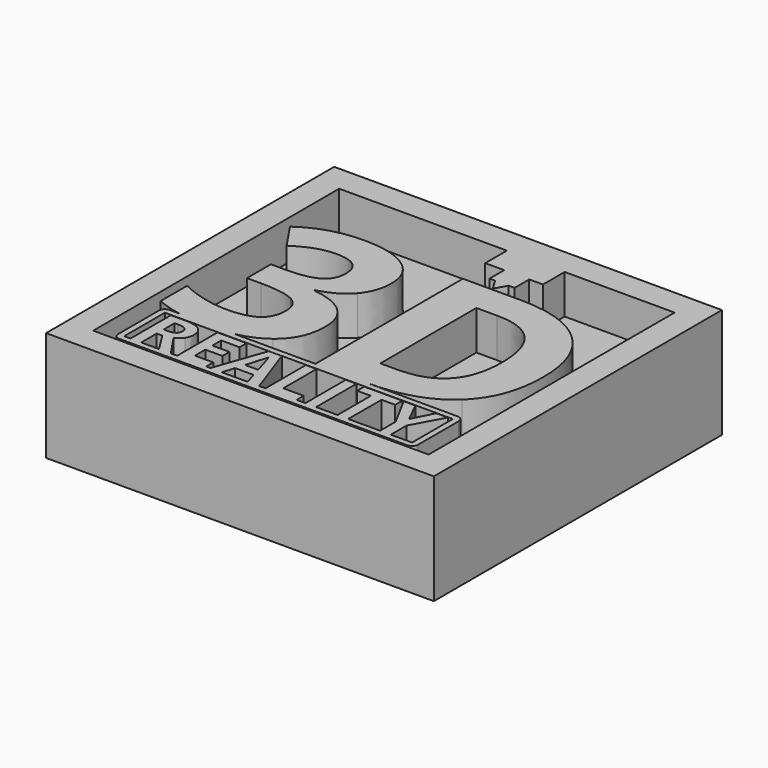
from build123d import *

# Parameters (mm, degrees)
F0_W     = 29.631577395
F0_H     = 27.5178048387
F1_DEPTH = 8.4
F3_DEPTH = 3
F4_SCALE = 2


# Not quite as in the source:
# - a feature names something its author has since deleted; it is built from what else it names


with BuildPart() as f1:
    # F0 (on Top) → F1 (new body)
    with BuildSketch(Plane.XY):
        with Locations((2.3732986487, -1.4568324946)):
            Rectangle(F0_W, F0_H)
    extrude(amount=F1_DEPTH)

    # F2 (on face) → F3 (cut)
    with BuildSketch(Plane.XY.offset(8.4)):
        Polygon((-10.4424900488, 10.2828489617), (-10.4424900488, -13.2157349139), (15.1890873462, -13.2157349139), (15.1890873462, 9.2640894619), (15.1890873462, 10.2828489617), (6.7861341126, 10.2828489617), (6.7861341126, 8.2122515887), (5.7374828029, 8.2122515887), (5.7374828029, 6.8167368881), (5.2872577988, 6.8167368881), (4.7797049629, 5.9268257703), (4.2468055268, 6.8167368881), (3.8219271228, 6.8167368881), (3.8219271228, 8.2122515887), (2.3732986487, 8.2122515887), (2.3732986487, 10.2828489617), align=None)
        with BuildLine():
            ThreePointArc((13.4450163236, -8.2785334899), (13.7646569396, -8.410090613), (13.8990873462, -8.7285334899))
            Line((13.8990873462, -8.7285334899), (13.8990873462, -12.6163954266))
            ThreePointArc((13.8990873462, -12.6163954266), (13.7646569396, -12.9348383034), (13.4450163236, -13.0663954266))
            Line((13.4450163236, -13.0663954266), (-8.5549836764, -13.0663954266))
            ThreePointArc((-8.5549836764, -13.0663954266), (-8.8731817279, -12.9345934781), (-9.0049836764, -12.6163954266))
            Line((-9.0049836764, -12.6163954266), (-9.0049836764, -8.7285334899))
            ThreePointArc((-9.0049836764, -8.7285334899), (-8.8731817279, -8.4103354383), (-8.5549836764, -8.2785334899))
            Line((-8.5549836764, -8.2785334899), (-7.8079242079, -8.2785334899))
            add(Edge.make_bspline(
                [(-7.8079242079, -8.2785334899), (-8.8129286115, -8.0881923504), (-9.6902965463, -7.7113056027)],
                knots=[0.5050353738, 0.5050353738, 0.5050353738, 1, 1, 1], degree=2))
            Line((-9.6902965463, -7.7113056027), (-9.6902965463, -5.1772766722))
            add(Edge.make_bspline(
                [(-9.6902965463, -5.1772766722), (-8.8733650784, -5.5903665465), (-7.8899645568, -5.8508597882)],
                knots=[0, 0, 0, 1, 1, 1], degree=2))
            add(Edge.make_bspline(
                [(-7.8899645568, -5.8508597882), (-6.9065640351, -6.1113530298), (-5.9447428351, -6.1113530298)],
                knots=[0, 0, 0, 1, 1, 1], degree=2))
            add(Edge.make_bspline(
                [(-5.9447428351, -6.1113530298), (-4.4681006725, -6.1113530298), (-3.7652313341, -5.6104044882)],
                knots=[0, 0, 0, 1, 1, 1], degree=2))
            add(Edge.make_bspline(
                [(-3.7652313341, -5.6104044882), (-3.0623619957, -5.1094559466), (-3.0623619957, -3.9996622544)],
                knots=[0, 0, 0, 1, 1, 1], degree=2))
            add(Edge.make_bspline(
                [(-3.0623619957, -3.9996622544), (-3.0623619957, -3.0100962122), (-3.8715865629, -2.5954649577)],
                knots=[0, 0, 0, 1, 1, 1], degree=2))
            add(Edge.make_bspline(
                [(-3.8715865629, -2.5954649577), (-4.6808111301, -2.1808337033), (-6.4533982774, -2.1808337033)],
                knots=[0, 0, 0, 1, 1, 1], degree=2))
            Line((-6.4533982774, -2.1808337033), (-7.5231160863, -2.1808337033))
            Line((-7.5231160863, -2.1808337033), (-7.5231160863, 0.1034916465))
            Line((-7.5231160863, 0.1034916465), (-6.4349017159, 0.1034916465))
            add(Edge.make_bspline(
                [(-6.4349017159, 0.1034916465), (-4.7979560199, 0.1034916465), (-4.041138377, 0.5319953221)],
                knots=[0, 0, 0, 1, 1, 1], degree=2))
            add(Edge.make_bspline(
                [(-4.041138377, 0.5319953221), (-3.2843207341, 0.9604989977), (-3.2843207341, 1.999389204)],
                knots=[0, 0, 0, 1, 1, 1], degree=2))
            add(Edge.make_bspline(
                [(-3.2843207341, 1.999389204), (-3.2843207341, 3.5993417769), (-5.2881149006, 3.5993417769)],
                knots=[0, 0, 0, 1, 1, 1], degree=2))
            add(Edge.make_bspline(
                [(-5.2881149006, 3.5993417769), (-5.9817359582, 3.5993417769), (-6.7000190979, 3.3681347577)],
                knots=[0, 0, 0, 1, 1, 1], degree=2))
            add(Edge.make_bspline(
                [(-6.7000190979, 3.3681347577), (-7.4183022376, 3.1369277385), (-8.2938061503, 2.5696998514)],
                knots=[0, 0, 0, 1, 1, 1], degree=2))
            Line((-8.2938061503, 2.5696998514), (-9.6717999848, 4.6197354217))
            add(Edge.make_bspline(
                [(-9.6717999848, 4.6197354217), (-7.7450748247, 6.0069775369), (-5.0754044429, 6.0069775369)],
                knots=[0, 0, 0, 1, 1, 1], degree=2))
            add(Edge.make_bspline(
                [(-5.0754044429, 6.0069775369), (-2.8897274213, 6.0069775369), (-1.6227129561, 5.1206839633)],
                knots=[0, 0, 0, 1, 1, 1], degree=2))
            add(Edge.make_bspline(
                [(-1.6227129561, 5.1206839633), (-0.3556984908, 4.2343903897), (-0.3556984908, 2.6560171385)],
                knots=[0, 0, 0, 1, 1, 1], degree=2))
            add(Edge.make_bspline(
                [(-0.3556984908, 2.6560171385), (-0.3556984908, 1.3365957489), (-1.1556747773, 0.4117676721)],
                knots=[0, 0, 0, 1, 1, 1], degree=2))
            add(Edge.make_bspline(
                [(-1.1556747773, 0.4117676721), (-1.9556510637, -0.5130604047), (-3.4014656239, -0.8614123137)],
                knots=[0, 0, 0, 1, 1, 1], degree=2))
            Line((-3.4014656239, -0.8614123137), (-3.4014656239, -0.9169019983))
            add(Edge.make_bspline(
                [(-3.4014656239, -0.9169019983), (-1.693616442, -1.129612456), (-0.8181125292, -1.9542508245)],
                knots=[0, 0, 0, 1, 1, 1], degree=2))
            add(Edge.make_bspline(
                [(-0.8181125292, -1.9542508245), (0.0573913835, -2.778889193), (0.0573913835, -4.175379589)],
                knots=[0, 0, 0, 1, 1, 1], degree=2))
            add(Edge.make_bspline(
                [(0.0573913835, -4.175379589), (0.0573913835, -6.2069185978), (-1.4161680189, -7.3398329919)],
                knots=[0, 0, 0, 1, 1, 1], degree=2))
            add(Edge.make_bspline(
                [(-1.4161680189, -7.3398329919), (-2.2796158654, -8.003676263), (-3.5759760712, -8.2785334899)],
                knots=[0, 0, 0, 0.5859606644, 0.5859606644, 0.5859606644], degree=2))
            Line((-3.5759760712, -8.2785334899), (2.591420314, -8.2785334899))
            Line((2.591420314, -8.2785334899), (2.591420314, 5.8065981203))
            Line((2.591420314, 5.8065981203), (7.0120985213, 5.8065981203))
            add(Edge.make_bspline(
                [(7.0120985213, 5.8065981203), (10.4617072478, 5.8065981203), (12.3699358464, 3.9862281891)],
                knots=[0, 0, 0, 1, 1, 1], degree=2))
            add(Edge.make_bspline(
                [(12.3699358464, 3.9862281891), (14.2781644449, 2.1658582578), (14.2781644449, -1.1018676137)],
                knots=[0, 0, 0, 1, 1, 1], degree=2))
            add(Edge.make_bspline(
                [(14.2781644449, -1.1018676137), (14.2781644449, -4.5792211825), (12.2974909804, -6.4288773362)],
                knots=[0, 0, 0, 1, 1, 1], degree=2))
            add(Edge.make_bspline(
                [(12.2974909804, -6.4288773362), (10.3168175158, -8.2785334899), (6.5805120854, -8.2785334899)],
                knots=[0, 0, 0, 1, 1, 1], degree=2))
            Line((6.5805120854, -8.2785334899), (13.4450163236, -8.2785334899))
        make_face(mode=Mode.SUBTRACT)
        with BuildLine():
            add(Edge.make_bspline(
                [(6.8579605085, -5.812325285), (11.173824867, -5.812325285), (11.173824867, -1.1789366201)],
                knots=[0, 0, 0, 1, 1, 1], degree=2))
            add(Edge.make_bspline(
                [(11.173824867, -1.1789366201), (11.173824867, 3.3588864769), (7.1662365341, 3.3588864769)],
                knots=[0, 0, 0, 1, 1, 1], degree=2))
            Line((7.1662365341, 3.3588864769), (5.5786150022, 3.3588864769))
            Line((5.5786150022, 3.3588864769), (5.5786150022, -5.812325285))
            Line((5.5786150022, -5.812325285), (6.8579605085, -5.812325285))
        make_face()
        with BuildLine():
            Line((13.4450163236, -8.7285334899), (-8.5549836764, -8.7285334899))
            Line((-8.5549836764, -8.7285334899), (-8.5549836764, -12.6163954266))
            Line((-8.5549836764, -12.6163954266), (-8.0698446543, -12.6163954266))
            Line((-8.0698446543, -12.6163954266), (-8.0698446543, -8.7614385714))
            Line((-8.0698446543, -8.7614385714), (-6.9468532833, -8.7614385714))
            add(Edge.make_bspline(
                [(-6.9468532833, -8.7614385714), (-6.1605062075, -8.7614385714), (-5.7837852104, -9.0474596644)],
                knots=[0, 0, 0, 1, 1, 1], degree=2))
            add(Edge.make_bspline(
                [(-5.7837852104, -9.0474596644), (-5.4070642133, -9.3334807574), (-5.4070642133, -9.9164913039)],
                knots=[0, 0, 0, 1, 1, 1], degree=2))
            add(Edge.make_bspline(
                [(-5.4070642133, -9.9164913039), (-5.4070642133, -10.2565104793), (-5.5939482018, -10.5214385714)],
                knots=[0, 0, 0, 1, 1, 1], degree=2))
            add(Edge.make_bspline(
                [(-5.5939482018, -10.5214385714), (-5.7808321903, -10.7863666634), (-6.1242262459, -10.9365488302)],
                knots=[0, 0, 0, 1, 1, 1], degree=2))
            add(Edge.make_bspline(
                [(-6.1242262459, -10.9365488302), (-5.2535071663, -12.2367214093), (-4.9902665143, -12.6163954266)],
                knots=[0, 0, 0, 1, 1, 1], degree=2))
            Line((-4.9902665143, -12.6163954266), (-4.5051274923, -12.6163954266))
            Line((-4.5051274923, -12.6163954266), (-4.5051274923, -8.7614385714))
            Line((-4.5051274923, -8.7614385714), (-2.2853000714, -8.7614385714))
            Line((-2.2853000714, -8.7614385714), (-2.2853000714, -9.4313522818))
            Line((-2.2853000714, -9.4313522818), (-3.6875627751, -9.4313522818))
            Line((-3.6875627751, -9.4313522818), (-3.6875627751, -10.2776034803))
            Line((-3.6875627751, -10.2776034803), (-2.3823278758, -10.2776034803))
            Line((-2.3823278758, -10.2776034803), (-2.3823278758, -10.9475171907))
            Line((-2.3823278758, -10.9475171907), (-3.6875627751, -10.9475171907))
            Line((-3.6875627751, -10.9475171907), (-3.6875627751, -11.9414193959))
            Line((-3.6875627751, -11.9414193959), (-2.2853000714, -11.9414193959))
            Line((-2.2853000714, -11.9414193959), (-2.2853000714, -12.6163954266))
            Line((-2.2853000714, -12.6163954266), (-1.9663738969, -12.6163954266))
            Line((-1.9663738969, -12.6163954266), (-0.605453475, -8.7454078906))
            Line((-0.605453475, -8.7454078906), (0.3935110504, -8.7454078906))
            Line((0.3935110504, -8.7454078906), (1.7594937925, -12.6163954266))
            Line((1.7594937925, -12.6163954266), (2.2446328145, -12.6163954266))
            Line((2.2446328145, -12.6163954266), (2.2446328145, -8.7614385714))
            Line((2.2446328145, -8.7614385714), (3.0621975317, -8.7614385714))
            Line((3.0621975317, -8.7614385714), (3.0621975317, -11.9414193959))
            Line((3.0621975317, -11.9414193959), (4.6256107627, -11.9414193959))
            Line((4.6256107627, -11.9414193959), (4.6256107627, -12.6163954266))
            Line((4.6256107627, -12.6163954266), (5.2955244732, -12.6163954266))
            Line((5.2955244732, -12.6163954266), (5.2955244732, -8.7614385714))
            Line((5.2955244732, -8.7614385714), (6.1130891904, -8.7614385714))
            Line((6.1130891904, -8.7614385714), (6.1130891904, -12.6163954266))
            Line((6.1130891904, -12.6163954266), (7.7532809449, -12.6163954266))
            Line((7.7532809449, -12.6163954266), (7.7532809449, -9.4414769223))
            Line((7.7532809449, -9.4414769223), (6.7062243773, -9.4414769223))
            Line((6.7062243773, -9.4414769223), (6.7062243773, -8.7614385714))
            Line((6.7062243773, -8.7614385714), (9.6170585096, -8.7614385714))
            Line((9.6170585096, -8.7614385714), (9.6170585096, -9.4414769223))
            Line((9.6170585096, -9.4414769223), (8.5708456621, -9.4414769223))
            Line((8.5708456621, -9.4414769223), (8.5708456621, -12.6163954266))
            Line((8.5708456621, -12.6163954266), (11.0041342527, -12.6163954266))
            Line((11.0041342527, -12.6163954266), (11.0041342527, -11.1424165196))
            Line((11.0041342527, -11.1424165196), (9.7250546745, -8.7614385714))
            Line((9.7250546745, -8.7614385714), (10.6109607148, -8.7614385714))
            Line((10.6109607148, -8.7614385714), (11.4099635911, -10.3484759635))
            Line((11.4099635911, -10.3484759635), (12.2140287877, -8.7614385714))
            Line((12.2140287877, -8.7614385714), (13.0948725077, -8.7614385714))
            Line((13.0948725077, -8.7614385714), (11.8157929296, -11.1162611984))
            Line((11.8157929296, -11.1162611984), (11.8157929296, -12.6163954266))
            Line((11.8157929296, -12.6163954266), (13.4450163236, -12.6163954266))
            Line((13.4450163236, -12.6163954266), (13.4450163236, -8.7285334899))
        make_face()
        Polygon((-0.8062588442, -11.6984280249), (-1.0855301769, -12.6163954266), (0.8786500724, -12.6163954266), (0.5993787397, -11.6984280249), align=None)
        with BuildLine():
            Line((-0.6003911548, -11.0133273537), (0.4036356908, -11.0133273537))
            add(Edge.make_bspline(
                [(0.4036356908, -11.0133273537), (0.0163681932, -9.766309137), (-0.032567569, -9.6026274496)],
                knots=[0, 0, 0, 1, 1, 1], degree=2))
            add(Edge.make_bspline(
                [(-0.032567569, -9.6026274496), (-0.0815033312, -9.4389457622), (-0.1025963322, -9.3444491179)],
                knots=[0, 0, 0, 1, 1, 1], degree=2))
            add(Edge.make_bspline(
                [(-0.1025963322, -9.3444491179), (-0.1894994961, -9.6819371332), (-0.6003911548, -11.0133273537)],
                knots=[0, 0, 0, 1, 1, 1], degree=2))
        make_face()
        with BuildLine():
            Line((-7.2522799372, -9.4313522818), (-7.2522799372, -10.4725028091))
            Line((-7.2522799372, -10.4725028091), (-6.9890392852, -10.4725028091))
            add(Edge.make_bspline(
                [(-6.9890392852, -10.4725028091), (-6.6009280676, -10.4725028091), (-6.4165752392, -10.3434136433)],
                knots=[0, 0, 0, 1, 1, 1], degree=2))
            add(Edge.make_bspline(
                [(-6.4165752392, -10.3434136433), (-6.2322224108, -10.2143244774), (-6.2322224108, -9.9375843048)],
                knots=[0, 0, 0, 1, 1, 1], degree=2))
            add(Edge.make_bspline(
                [(-6.2322224108, -9.9375843048), (-6.2322224108, -9.6633752924), (-6.4207938394, -9.5473637871)],
                knots=[0, 0, 0, 1, 1, 1], degree=2))
            add(Edge.make_bspline(
                [(-6.4207938394, -9.5473637871), (-6.6093652679, -9.4313522818), (-7.0042262459, -9.4313522818)],
                knots=[0, 0, 0, 1, 1, 1], degree=2))
            Line((-7.0042262459, -9.4313522818), (-7.2522799372, -9.4313522818))
        make_face()
        Polygon((-7.2522799372, -11.1373541994), (-7.2522799372, -12.6163954266), (-5.8972655556, -12.6163954266), (-6.8177641174, -11.1373541994), align=None)
    extrude(amount=-F3_DEPTH, mode=Mode.SUBTRACT)


with BuildPart() as f1_1:
    # F4: moved
    add(f1.part.scale(F4_SCALE).moved(Location((12.4424900488, 15.2157349139, 0))))


solid = f1_1.part
